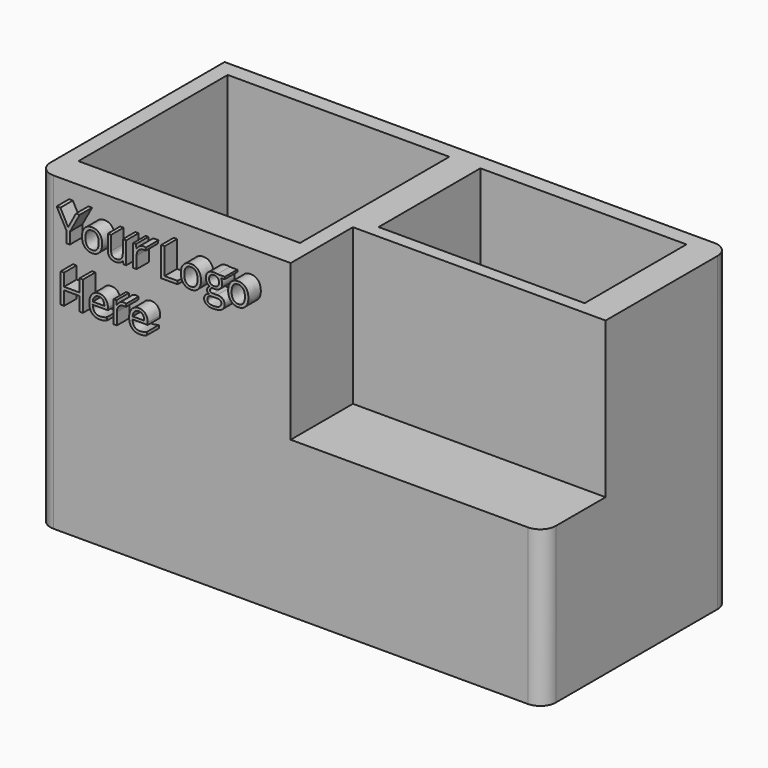
from build123d import *

# Parameters (mm, degrees)
F0_W         = 65
F0_H         = 30
F1_DEPTH     = 40
F2_W         = 32.5
F2_H         = 20
F3_DEPTH     = 10
F4_R         = 2
F5_W         = 28.5
F5_H         = 24
F6_DEPTH     = 35
F5_W_2       = 26.5
F5_H_2       = 16.3662411012
F7_DEPTH     = 35
F8_TEXT_SIZE = 5.2859361062
F9_DEPTH     = 2


# Not quite as in the source:
# - Text() gives the source's letters only with a copy of the font that has no kerning and outlines rounded to 1/6400 em; it was checked with that copy


with BuildPart() as f1:
    # F0 (on Top) → F1 (new body)
    with BuildSketch(Plane.XY):
        with Locations((6.5317551792, -0.7892294228)):
            Rectangle(F0_W, F0_H)
    extrude(amount=F1_DEPTH)

    # F2 (on face) → F3 (cut)
    with BuildSketch(Plane.XZ.offset(15.7892294228)):
        with Locations((22.7817551792, 30)):
            Rectangle(F2_W, F2_H)
    extrude(amount=-F3_DEPTH, mode=Mode.SUBTRACT)

    # F4
    f4_edges = [f1.edges().sort_by_distance(p)[0] for p in [
        (39.031755, -15.789229, 10),
        (39.031755, 14.210771, 20),
        (-25.968245, -15.789229, 20),
    ]]
    fillet(f4_edges, radius=F4_R)

    # F5 (on face) → F6 (cut)
    with BuildSketch(Plane.XY.offset(40)):
        with Locations((-9.7182448208, 0.2107705772)):
            Rectangle(F5_W, F5_H)
    extrude(amount=-F6_DEPTH, mode=Mode.SUBTRACT)

    # F5 (on face) → F7 (cut)
    with BuildSketch(Plane.XY.offset(40)):
        with Locations((21.7817551792, 4.0276500266)):
            Rectangle(F5_W_2, F5_H_2)
    extrude(amount=-F7_DEPTH, mode=Mode.SUBTRACT)

    # F8 (on face) → F9 (join)
    with BuildSketch(Plane.XZ.offset(15.7892294228)):
        with Locations((-21.9682448208, 34.1941260035)):
            Text('Your Logo', F8_TEXT_SIZE, font='Open Sans', text_align=(TextAlign.LEFT, TextAlign.BOTTOM))
        with Locations((-21.9682448208, 27.005252899)):
            Text('Here', F8_TEXT_SIZE, font='Open Sans', text_align=(TextAlign.LEFT, TextAlign.BOTTOM))
    extrude(amount=F9_DEPTH)


solid = f1.part
